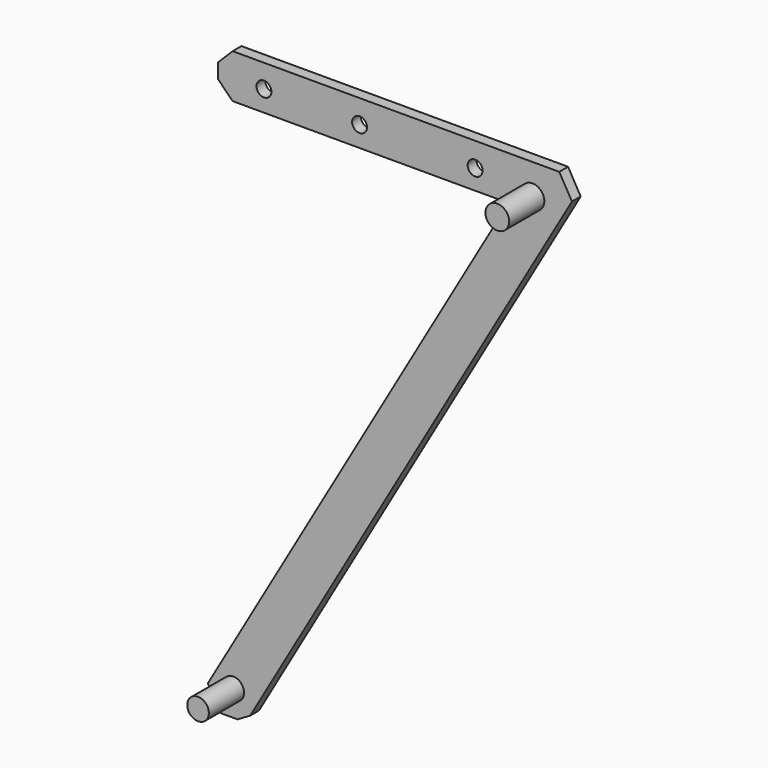
from build123d import *

# Parameters (mm, degrees)
F1_DEPTH    = 19.05
F3_DEPTH    = 19.05
F5_D        = 25.8064
F7_R        = 20.5102138496
F7_R_2      = 18.7123578019
F8_DEPTH    = 76.2
F9_T1_DEPTH = 149.6914957887
F9_T3_DEPTH = 96.8143860217
F9_T5_DEPTH = 241.603940201


# Not quite as in the source:
# - a fillet or chamfer that OpenCascade refuses, or shapes differently, is made with other operations: its cross-section is extruded or revolved along the edge and cut away or added


with BuildPart() as f1:
    # F0 (on Front) → F1 (new body)
    with BuildSketch(Plane.XZ):
        Polygon((315.2909820045, 546.1), (227.30280098, 546.1), (-359.2850725167, -469.9), (-271.2968914922, -469.9), align=None)
    extrude(amount=F1_DEPTH)

    # F2 (on face) → F3 (join, through all)
    with BuildSketch(Plane.XZ.offset(19.05)):
        Polygon((227.30280098, 546.1), (-319.7090179955, 546.1), (-319.7090179955, 469.9), (183.3087104677, 469.9), align=None)
    extrude(amount=-F3_DEPTH)

    # F5 (through all)
    with Locations(Plane.XZ.offset(19.05)):
        with Locations((-240.0867491961, 506.0059428215), (-74.4647756219, 505.5469870567), (125.6440877914, 504.5655369759)):
            Hole(F5_D / 2)

    # F7 (on offset) → F8 (join, through all)
    with BuildSketch(Plane.XZ.offset(95.25)):
        with Locations((224.993377924, 492.937207222)):
            Circle(F7_R)
        with Locations((-293.2454049587, -425.5582988262)):
            Circle(F7_R_2)
    extrude(amount=-F8_DEPTH)

    # F9: chamfer of 25.4 on 5 edges, made by hand

    # F9_s2 → F9_t1 (cut)
    with BuildSketch(Plane.XZ.offset(-65.3207478943)):
        Polygon((-294.3090179955, 546.1), (-319.7090179955, 520.7), (-319.7090179955, 546.1), align=None)
        Polygon((-294.3090179955, 469.9), (-319.7090179955, 495.3), (-319.7090179955, 469.9), align=None)
    extrude(amount=F9_T1_DEPTH, mode=Mode.SUBTRACT)

    # F9_s4 → F9_t3 (cut)
    with BuildSketch(Plane.XZ.offset(-38.8821930109)):
        Polygon((-285.9615883296, -469.9), (-263.9645430735, -457.2), (-271.2968914922, -469.9), align=None)
    extrude(amount=F9_T3_DEPTH, mode=Mode.SUBTRACT)

    # F9_s6 → F9_t5 (cut)
    with BuildSketch(Plane.XZ.offset(-111.2769701005)):
        Polygon((293.2939367483, 508), (271.2968914922, 546.1), (315.2909820045, 546.1), align=None)
        Polygon((-315.2909820045, -469.9), (-337.2880272606, -431.8), (-359.2850725167, -469.9), align=None)
    extrude(amount=F9_T5_DEPTH, mode=Mode.SUBTRACT)


solid = f1.part
